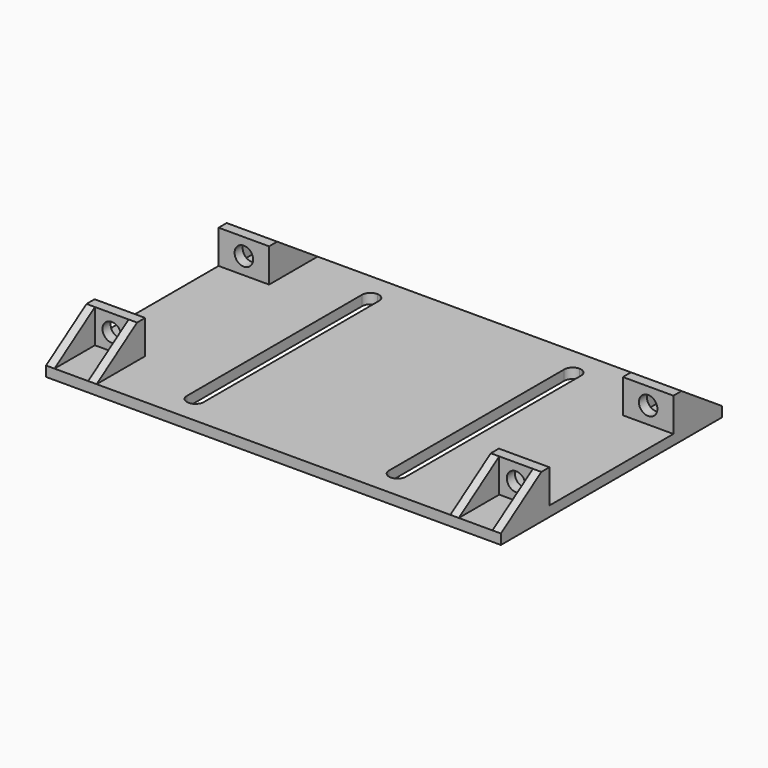
from build123d import *

# Parameters (mm, degrees)
F0_W      = 135
F0_H      = 82
F1_DEPTH  = 3
F2_W      = 3
F2_H      = 10
F3_DEPTH  = 15
F4_DEPTH  = 15
F5_W      = 10
F5_H      = 15
F6_DEPTH  = 25
F8_D      = 5.5
F8_DEPTH  = 10
F8_TIP    = 1.6523667023
F12_COUNT = 2


# Not quite as in the source:
# - a feature names something its author has since deleted; it is built from what else it names


with BuildPart() as f1:
    # F0 (on Top) → F1 (new body)
    with BuildSketch(Plane.XY):
        Rectangle(F0_W, F0_H)
        with BuildLine():
            Line((-32.5, -32.5), (-32.5, 32.5))
            ThreePointArc((-32.5, 32.5), (-31.767766953, 34.267766953), (-30, 35))
            ThreePointArc((-30, 35), (-28.232233047, 34.267766953), (-27.5, 32.5))
            Line((-27.5, 32.5), (-27.5, -32.5))
            ThreePointArc((-27.5, -32.5), (-28.232233047, -34.267766953), (-30, -35))
            ThreePointArc((-30, -35), (-31.767766953, -34.267766953), (-32.5, -32.5))
        make_face(mode=Mode.SUBTRACT)
        with BuildLine():
            Line((27.5, -32.5), (27.5, 32.5))
            ThreePointArc((27.5, 32.5), (28.232233047, 34.267766953), (30, 35))
            ThreePointArc((30, 35), (31.767766953, 34.267766953), (32.5, 32.5))
            Line((32.5, 32.5), (32.5, -32.5))
            ThreePointArc((32.5, -32.5), (31.767766953, -34.267766953), (30, -35))
            ThreePointArc((30, -35), (28.232233047, -34.267766953), (27.5, -32.5))
        make_face(mode=Mode.SUBTRACT)
    extrude(amount=F1_DEPTH)

    # F2 (on face) → F3 (join)
    with BuildSketch(Plane.YZ.offset(67.5)):
        with Locations((-24.5, 8)):
            Rectangle(F2_W, F2_H)
    extrude(amount=-F3_DEPTH)

    # F2 (on face) → F4 (join)
    with BuildSketch(Plane.YZ.offset(67.5)):
        Polygon((-41, 3), (-26, 3), (-26, 13), align=None)
    extrude(amount=-F4_DEPTH)

    # F5 (on face) → F6 (cut)
    with BuildSketch(Plane.XY.offset(3)):
        with Locations((60, -33.5)):
            Rectangle(F5_W, F5_H)
    extrude(amount=F6_DEPTH, mode=Mode.SUBTRACT)

    # F8
    with Locations(Plane(origin=(0, -23, 0), x_dir=(-1, 0, 0), z_dir=(0, 1, 0))):
        with Locations((-60, 8)):
            Hole(F8_D / 2, depth=F8_DEPTH)
            with Locations((0, 0, -(F8_DEPTH + F8_TIP / 2))):  # 118° drill point
                Cone(0, F8_D / 2, F8_TIP, mode=Mode.SUBTRACT)

    # F10: F1 across plane


with BuildPart() as f1_1:
    add(f1.part)
    add(f1.part.mirror(Plane.YZ))

    # F12: F1 ×2 about axis
    f12_axis = Axis((0, 0, 10.3634241968), (0, 0, -1))


with BuildPart() as f1_2:
    add(f1_1.part)
    for i in range(1, F12_COUNT):
        add(f1_1.part.rotate(f12_axis, i * 360 / F12_COUNT))


solid = f1_2.part
